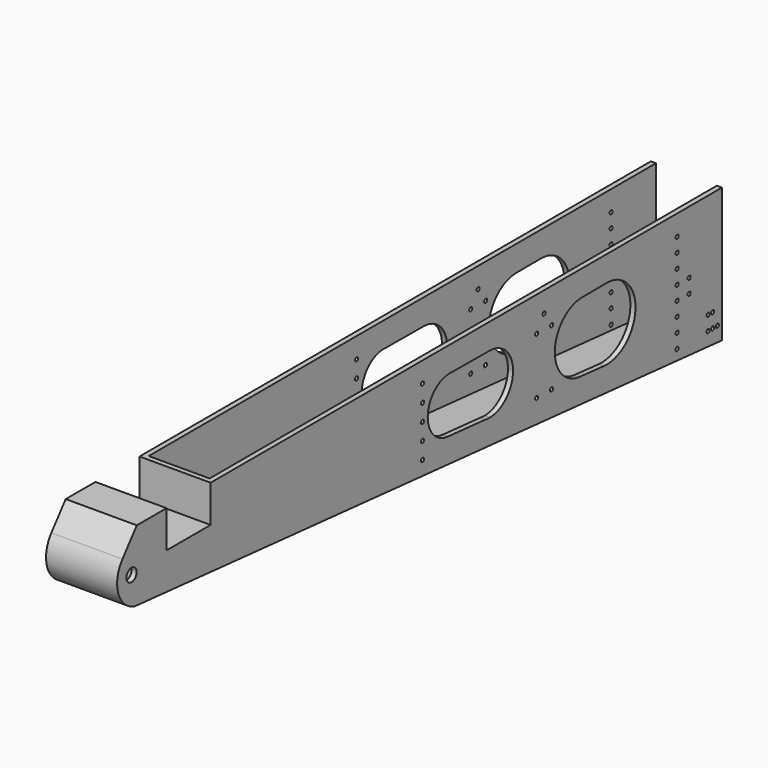
from build123d import *

# Parameters (mm, degrees)
F1_DEPTH    = 55.5
F2_T        = 4
F2_T3_DEPTH = 63.5
F3_R        = 1.5
F3_R_2      = 5
F4_DEPTH    = 132
F6_START    = -4
F6_DEPTH    = 47.5


# Not quite as in the source:
# - a shell that OpenCascade refuses in one call is made with other operations: the cavity is built on its own and cut out


with BuildPart() as f1:
    # F0 (on Right) → F1 (new body)
    with BuildSketch(Plane.YZ):
        with BuildLine():
            Line((0, -55.0991142094), (0, 49.9008857906))
            Line((0, 49.9008857906), (-499, 49.9008857906))
            Line((-499, 49.9008857906), (-499, 20.9008857906))
            Line((-499, 20.9008857906), (-542, 20.9008857906))
            Line((-542, 20.9008857906), (-542, 49.9008857906))
            Line((-542, 49.9008857906), (-571, 49.9008857906))
            Line((-571, 49.9008857906), (-585.0227475166, 32.4236936867))
            ThreePointArc((-585.0227475166, 32.4236936867), (-589.1305886162, 10.6178817454), (-573.3100487518, -4.9409842581))
            Line((-573.3100487518, -4.9409842581), (0, -55.0991142094))
        make_face()
        with BuildLine():
            ThreePointArc((-267.5215016214, -12.4960653082), (-287.1014882349, 8.865775765), (-267.5215016214, 30.2276168381))
            ThreePointArc((-267.5215016214, 30.2276168381), (-265.5317159892, 30.3083194328), (-263.5430244658, 30.2040803041))
            Line((-263.5430244658, 30.2040803041), (-227.1501212267, 29.9887811395))
            ThreePointArc((-227.1501212267, 29.9887811395), (-226.7168570765, 29.9902909304), (-226.2836411156, 29.983655073))
            ThreePointArc((-226.2836411156, 29.983655073), (-210.3577454889, 23.0383320758), (-203.8081448594, 6.9456506758))
            ThreePointArc((-203.8081448594, 6.9456506758), (-210.3577454889, -9.1470307242), (-226.2836411156, -16.0923537213))
            ThreePointArc((-226.2836411156, -16.0923537213), (-228.8553111139, -16.012257226), (-231.40202441, -15.6459876318))
            Line((-231.40202441, -15.6459876318), (-267.5215016214, -12.4960653082))
        make_face(mode=Mode.SUBTRACT)
        with BuildLine():
            ThreePointArc((-112.6117591226, 30.1063306123), (-92.6236860119, 21.9492705288), (-84.3273722818, 2.0185938124))
            ThreePointArc((-84.3273722818, 2.0185938124), (-93.5072337014, -18.7521971721), (-115.0464908191, -25.9463626291))
            Line((-115.0464908191, -25.9463626291), (-137.5543760441, -23.8290179612))
            ThreePointArc((-137.5543760441, -23.8290179612), (-138.6707155639, -23.7473709318), (-139.7826970584, -23.6193970408))
            ThreePointArc((-139.7826970584, -23.6193970408), (-163.0572812206, 4.0202298169), (-137.871291965, 29.9300963926))
            ThreePointArc((-137.871291965, 29.9300963926), (-136.3367885283, 29.9845849808), (-134.8016741863, 29.9515129286))
            Line((-134.8016741863, 29.9515129286), (-112.6117591226, 30.1063306123))
        make_face(mode=Mode.SUBTRACT)
    extrude(amount=F1_DEPTH)

    # F2: shell of thickness 4, made by hand


with BuildPart() as f2_core1:
    # F2_t2: copy of F1
    add(f1.part)

    # the walls: a layer under each face that stays
    f2_faces = [f2_core1.faces().sort_by_distance(p)[0] for p in [
        (55.5, -295.1049872852, -2.5991142094),
        (27.75, -163.0392168361, 4.4361103036),
        (27.75, -126.3004334316, -24.8876902951),
        (27.75, -84.3538324473, 0.7996810334),
        (27.75, -123.7067166544, 30.0289217705),
        (27.75, -203.9075264936, 4.8077471556),
        (27.75, -245.3465728463, 30.0964307218),
        (27.75, -287.0090157551, 10.8550491528),
        (27.75, -249.4617630157, -14.07102647),
        (27.75, -589.1305886162, 10.6178817454),
        (27.75, -578.0113737583, 41.1622897387),
        (27.75, -556.5, 49.9008857906),
        (27.75, -520.5, 20.9008857906),
        (27.75, -499, 35.4008857906),
        (0, -295.1049872852, -2.5991142094),
        (27.75, -286.6550243759, -30.0200492338),
    ]]
    thicken(f2_faces, amount=-F2_T, mode=Mode.SUBTRACT)

    # F2_s4 → F2_t3 (cut)
    with BuildSketch(Plane.YZ.offset(-4)):
        Polygon((-499.04, 20.9408857906), (-499, 16.9008857906), (-495, 16.9008857906), (-495, 20.9008857906), align=None)
    extrude(amount=F2_T3_DEPTH, mode=Mode.SUBTRACT)


with BuildPart() as f1_1:
    add(f1.part)

    # what is left inside the walls is the cavity
    f2_cavity = [f2_core1.part.solids().sort_by_distance(p)[0] for p in [
        (51.46, -293.104987, -17.422261),
    ]]
    add(f2_cavity, mode=Mode.SUBTRACT)

    # F3 (on face) → F4 (cut)
    with BuildSketch(Plane.YZ.offset(55.5)):
        with Locations((-43.75, 33.9008857906)):
            Circle(F3_R)
        with Locations((-43.75, 22.9008857906)):
            Circle(F3_R)
        with Locations((-43.75, 11.9008857906)):
            Circle(F3_R)
        with Locations((-43.75, 0.9008857906)):
            Circle(F3_R)
        with Locations((-43.75, -10.0991142094)):
            Circle(F3_R)
        with Locations((-43.75, -21.0991142094)):
            Circle(F3_R)
        with Locations((-43.75, -43.2409264798)):
            Circle(F3_R)
        with Locations((-43.75, -32.0991142094)):
            Circle(F3_R)
        with Locations((-32, 0.9008857906)):
            Circle(F3_R)
        with Locations((-32, -10.0991142094)):
            Circle(F3_R)
        with Locations((-4.5, -43.2409264798)):
            Circle(F3_R)
        with Locations((-9, -43.2409264798)):
            Circle(F3_R)
        with Locations((-9, -32.0991142094)):
            Circle(F3_R)
        with Locations((-13.5, -32.0991142094)):
            Circle(F3_R)
        with Locations((-13.5, -43.2409264798)):
            Circle(F3_R)
        with Locations((-166.25, -21.1966199487)):
            Circle(F3_R)
        with Locations((-180.75, 22.9008857906)):
            Circle(F3_R)
        with Locations((-180.75, -21.2039937677)):
            Circle(F3_R)
        with Locations((-166.25, 22.9008857906)):
            Circle(F3_R)
        with Locations((-173.5, 33.9008857906)):
            Circle(F3_R)
        with Locations((-292.1831863405, 33.9008857906)):
            Circle(F3_R)
        with Locations((-292.1831863405, -18.4991142094)):
            Circle(F3_R)
        with Locations((-292.1831863405, 20.8008857906)):
            Circle(F3_R)
        with Locations((-292.1831863405, 7.7008857906)):
            Circle(F3_R)
        with Locations((-292.1831863405, -5.3991142094)):
            Circle(F3_R)
        with Locations((-576.1306285858, 17.892671749)):
            Circle(F3_R_2)
    extrude(amount=-F4_DEPTH, mode=Mode.SUBTRACT)

    # F5 (on face) → F6 (cut)
    with BuildSketch(Plane.YZ.offset(55.5).offset(F6_START)):
        Polygon((-77.8550534083, 42.2289334238), (-298.9033162594, 42.2289334238), (-298.9033162594, -20.6155626995), (-77.8550534083, -39.8928311294), align=None)
    extrude(amount=-F6_DEPTH, mode=Mode.SUBTRACT)


solid = f1_1.part
